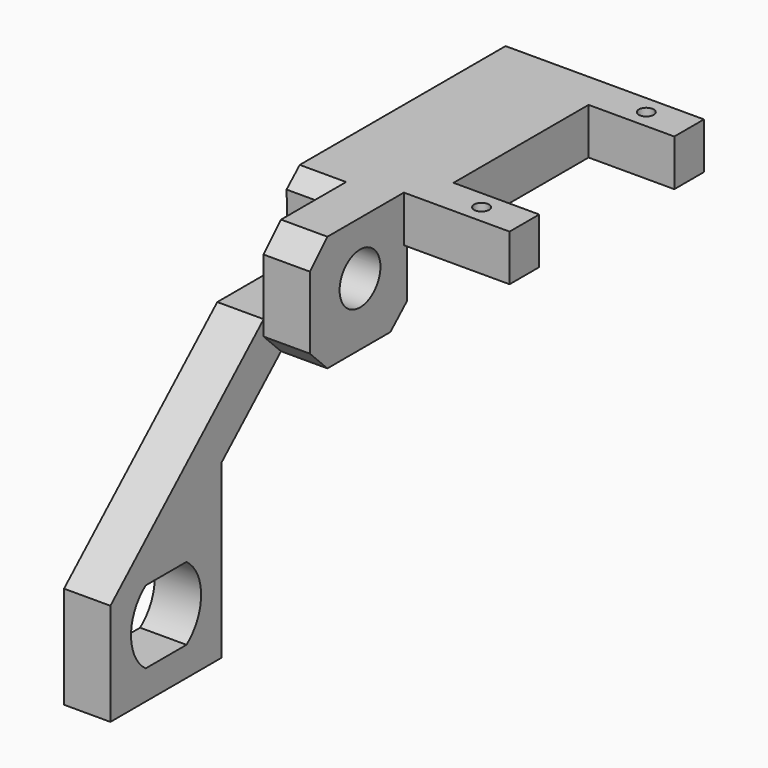
from build123d import *
from build123d import SkipClean  # not in build123d's __all__

# Parameters (mm, degrees)
F1_DEPTH = 6.35
F2_R     = 3.4925
F3_DEPTH = 6.35
F4_W     = 33.274
F4_H     = 6.35
F5_DEPTH = 9.08304
F6_W     = 5.08
F6_H     = 6.35
F7_DEPTH = 11.7348
F8_R     = 1.016
F9_DEPTH = 6.35


# Not quite as in the source:
# - after a boolean that leaves OpenCascade's solid faulty, fix() repairs it


with BuildPart() as f1:
    # F0 (on Right) → F1 (new body)
    with BuildSketch(Plane.YZ):
        with BuildLine():
            Line((0, -6.35), (0, 0))
            Line((0, 0), (-32.766, 0))
            Line((-32.766, 0), (-35.2239654818, 0))
            Line((-35.2239654818, 0), (-37.4816982729, -2.0558894312))
            Line((-37.4816982729, -2.0558894312), (-37.2950388694, -7.1750314139))
            ThreePointArc((-37.2950388694, -7.1750314139), (-38.2710574955, -9.7264527612), (-40.7852194514, -10.7947939567))
            Line((-40.7852194514, -10.7947939567), (-49.3363048096, -10.7947939567))
            Line((-49.3363048096, -10.7947939567), (-75.565, -34.67862))
            Line((-75.565, -34.67862), (-75.565, -48.67862))
            Line((-75.565, -48.67862), (-56.515, -48.67862))
            Line((-56.515, -48.67862), (-56.515, -25.1183178527))
            Line((-56.515, -25.1183178527), (-46.3639643027, -15.8747939567))
            Line((-46.3639643027, -15.8747939567), (-35.5806867418, -15.8747939567))
            Line((-35.5806867418, -15.8747939567), (-32.766, -13.3117427633))
            Line((-32.766, -13.3117427633), (-32.766, -6.35))
            Line((-32.766, -6.35), (0, -6.35))
        make_face()
        with BuildLine():
            ThreePointArc((-69.54, -44.67862), (-72.04, -39.67862), (-69.54, -34.67862))
            Line((-69.54, -34.67862), (-62.54, -34.67862))
            ThreePointArc((-62.54, -34.67862), (-60.04, -39.67862), (-62.54, -44.67862))
            Line((-62.54, -44.67862), (-69.54, -44.67862))
        make_face(mode=Mode.SUBTRACT)
    extrude(amount=F1_DEPTH)

    # F2 (on face) → F3 (join)
    with BuildSketch(Plane.YZ.offset(6.35)):
        Polygon((-32.766, -13.3117427633), (-32.766, 0), (-46.3639643027, 0), (-49.3577194514, -2.9937551487), (-49.3577194514, -12.8810388079), (-46.3639643027, -15.8747939567), (-35.5806867418, -15.8747939567), align=None)
        with Locations((-40.7852194514, -7.3022939567)):
            Circle(F2_R, mode=Mode.SUBTRACT)
    with SkipClean():  # cleaning this boolean's faces spoils the solid; the shape is the same uncleaned
        extrude(amount=F3_DEPTH)

    # F4 (on face) → F5 (join)
    with BuildSketch(Plane.YZ.offset(6.35)):
        with Locations((-16.637, -3.175)):
            Rectangle(F4_W, F4_H)
    extrude(amount=F5_DEPTH)

    add(f1.part.fix(), mode=Mode.REPLACE)

    # F6 (on face) → F7 (join)
    with BuildSketch(Plane.YZ.offset(15.43304)):
        with Locations((-2.54, -3.175)):
            Rectangle(F6_W, F6_H)
        with Locations((-30.734, -3.175)):
            Rectangle(F6_W, F6_H)
    extrude(amount=F7_DEPTH)

    add(f1.part.fix(), mode=Mode.REPLACE)

    # F8 (on face) → F9 (cut, through all)
    with BuildSketch(Plane.XY):
        with Locations((21.30044, -30.734)):
            Circle(F8_R)
        with Locations((21.30044, -2.54)):
            Circle(F8_R)
    extrude(amount=-F9_DEPTH, mode=Mode.SUBTRACT)


solid = f1.part
